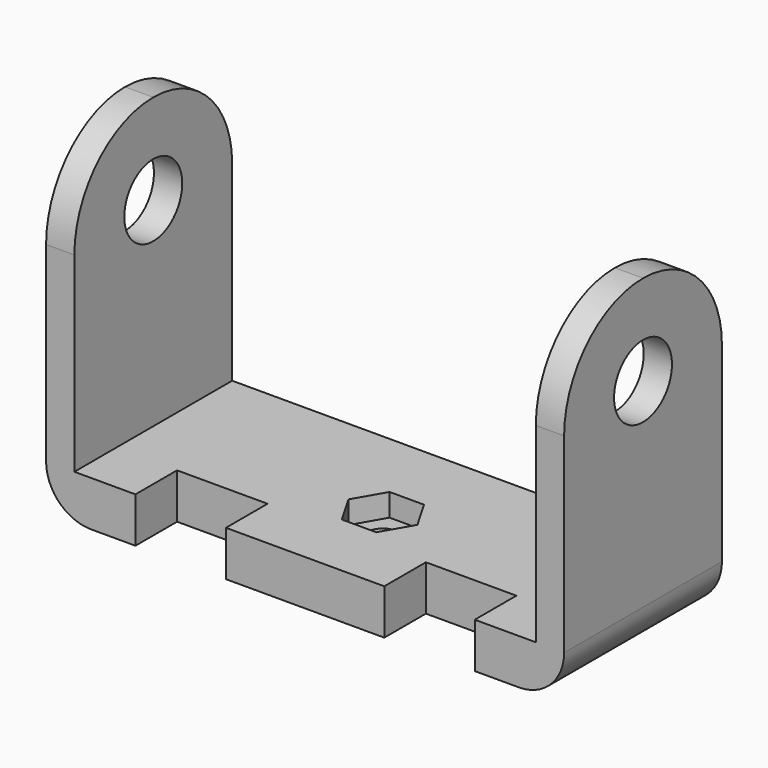
from build123d import *

# Parameters (mm, degrees)
F1_DEPTH       = 21.8
F2_R           = 4
F3_DEPTH       = 69.8
F4_R           = 10.89999
F5_W           = 10
F5_H           = 5.75
F5_H_2         = 0.9999994934
F6_DEPTH       = 25
F7_D           = 3.5
F7_DEPTH       = 10
F7_CSINK_D     = 5.5
F7_CSINK_ANGLE = 82
F7_TIP         = 1.0515060833
F8_R           = 1.75
F9_DEPTH       = 2.5
F10_R          = 5


# Not quite as in the source:
# - a fillet or chamfer is up to 0.001 mm smaller than in the source, because OpenCascade refuses the exact size


with BuildPart() as f1:
    # F0 (on Front) → F1 (new body)
    with BuildSketch(Plane.XZ):
        Polygon((-25.5, 37), (-28.625, 37), (-28.625, 0), (28.625, 0), (28.625, 37), (25.5, 37), (25.5, 5), (-25.5, 5), align=None)
    extrude(amount=F1_DEPTH)

    # F2 (on face) → F3 (cut)
    with BuildSketch(Plane(origin=(-28.625, 0, 0), x_dir=(0, -1, 0), z_dir=(-1, 0, 0))):
        with Locations((10.9, 27)):
            Circle(F2_R)
    extrude(amount=-F3_DEPTH, mode=Mode.SUBTRACT)

    # F4 (radius 10.9 in the source; OpenCascade refuses exactly that, so slightly less here)
    f4_edges = [f1.edges().sort_by_distance(p)[0] for p in [
        (-27.0625, -21.8, 37),
        (-27.0625, 0, 37),
        (27.0625, 0, 37),
        (27.0625, -21.8, 37),
    ]]
    fillet(f4_edges, radius=F4_R)

    # F5 (on face) → F6 (cut)
    with BuildSketch(Plane(origin=(0, 0, 0), x_dir=(1, 0, 0), z_dir=(0, 0, -1))):
        with Locations((-13.7500007451, 18.925)):
            Rectangle(F5_W, F5_H)
        with Locations((-13.7500007451, 22.2999997467)):
            Rectangle(F5_W, F5_H_2)
        with Locations((13.7500007451, 22.2999997467)):
            Rectangle(F5_W, F5_H_2)
        with Locations((13.7500007451, 18.925)):
            Rectangle(F5_W, F5_H)
    extrude(amount=-F6_DEPTH, mode=Mode.SUBTRACT)

    # F7
    with Locations(Plane(origin=(0, 0, 0), x_dir=(1, 0, 0), z_dir=(0, 0, -1))):
        with Locations((0, 11.05)):
            CounterSinkHole(F7_D / 2, F7_CSINK_D / 2, depth=F7_DEPTH, counter_sink_angle=F7_CSINK_ANGLE)
            with Locations((0, 0, -(F7_DEPTH + F7_TIP / 2))):  # 118° drill point
                Cone(0, F7_D / 2, F7_TIP, mode=Mode.SUBTRACT)

    # F8 (on face) → F9 (cut)
    with BuildSketch(Plane.XY.offset(5)):
        Polygon((1.9052558883, -7.75), (-1.9052558883, -7.75), (-3.8105117767, -11.05), (-1.9052558883, -14.35), (1.9052558883, -14.35), (3.8105117767, -11.05), align=None)
        with Locations((0, -11.05)):
            Circle(F8_R, mode=Mode.SUBTRACT)
    extrude(amount=-F9_DEPTH, mode=Mode.SUBTRACT)

    # F10
    f10_edges = [f1.edges().sort_by_distance(p)[0] for p in [
        (-28.625, -10.9, 0),
        (28.625, -10.9, 0),
    ]]
    fillet(f10_edges, radius=F10_R)


solid = f1.part
